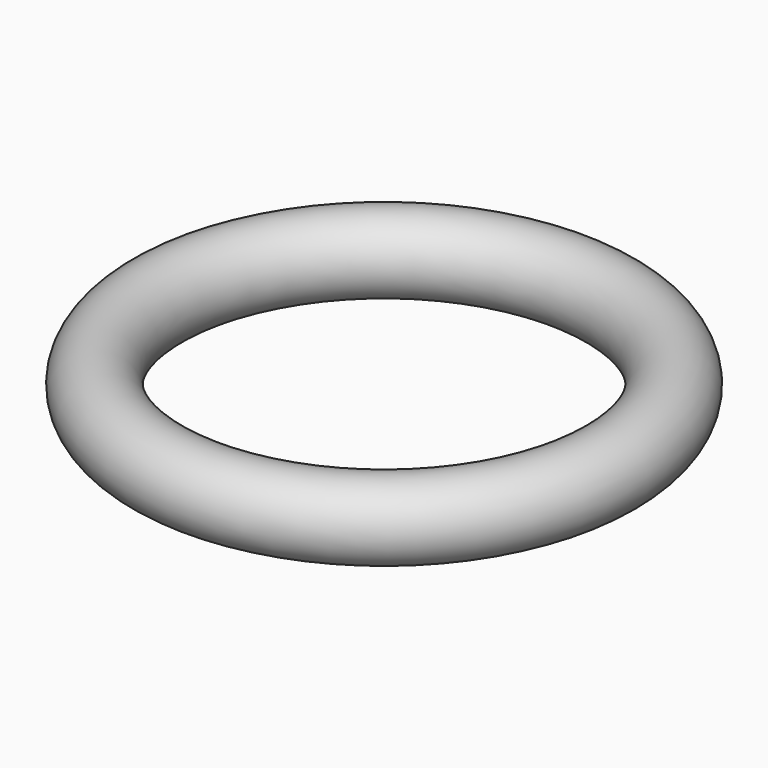
from build123d import *


# Not quite as in the source:
# - a feature of the source that left no trace in its solid (it failed there, or was rolled back) is left out


with BuildPart() as f1:
    # F0 (on Front) → F1 (revolve)
    with BuildSketch(Plane.XZ):
        with BuildLine():
            ThreePointArc((31.75, 9.9521605298), (38.1, 3.6021605298), (44.45, 9.9521605298))
            ThreePointArc((44.45, 9.9521605298), (38.1, 16.3021605298), (31.75, 9.9521605298))
        make_face()
    revolve(axis=Axis((0, 0, 0.1856796443), (0, 0, -1)))


solid = f1.part
